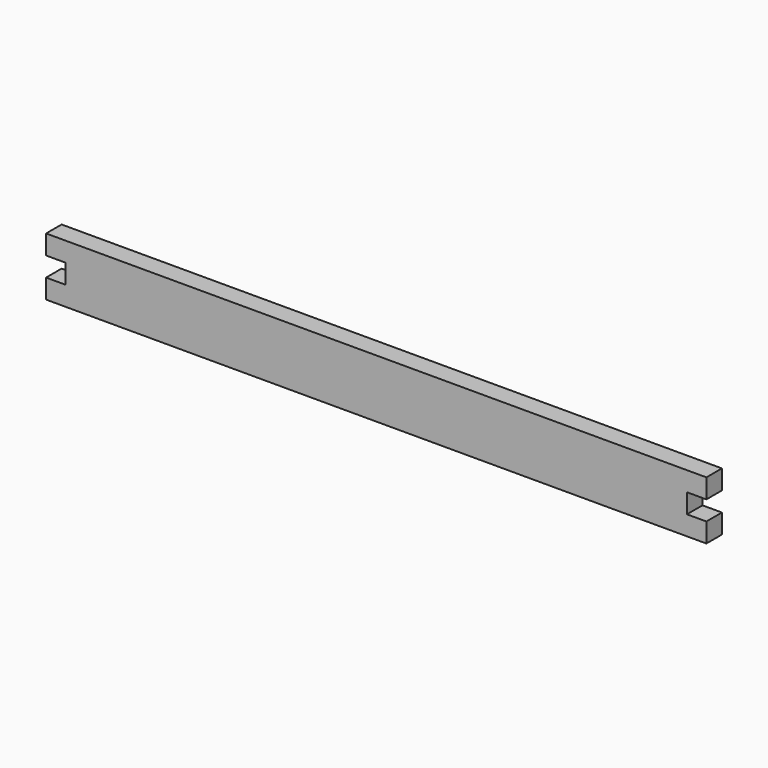
from build123d import *

# Parameters (mm, degrees)
F0_W     = 19.05
F0_H     = 19.05
F1_DEPTH = 19.05


# Not quite as in the source:
# - a feature names something its author has since deleted; it is built from what else it names


with BuildPart() as f1:
    # F0 (on Front) → F1 (new body)
    with BuildSketch(Plane.XZ):
        Polygon((312.9268772483, -147.6505908728), (-296.6731227517, -147.6505908728), (-315.7231227517, -147.6505908728), (-315.7231227517, -166.7005908728), (-296.6731227517, -166.7005908728), (-296.6731227517, -185.7505908728), (-315.7231227517, -185.7505908728), (-315.7231227517, -204.8005908728), (-296.6731227517, -204.8005908728), (312.9268772483, -204.8005908728), (312.9268772483, -185.7505908728), (312.9268772483, -166.7005908728), align=None)
        with Locations((322.4518772483, -157.1755908728)):
            Rectangle(F0_W, F0_H)
        with Locations((322.4518772483, -195.2755908728)):
            Rectangle(F0_W, F0_H)
    extrude(amount=F1_DEPTH)


solid = f1.part
